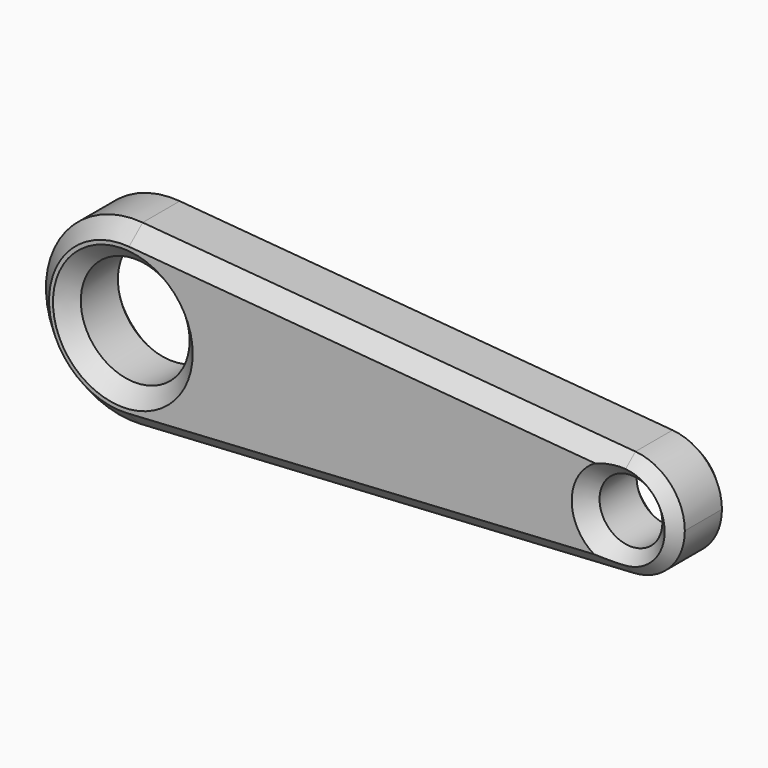
from build123d import *

# Parameters (mm, degrees)
F0_R         = 17.8816960504
F0_R_2       = 10.3302818728
F1_DEPTH     = 25.4
F2_T1_DEPTH  = 162.5438125483
F2_T3_DEPTH  = 162.5438125483
F2_T6_ANGLE  = 188.1812058846
F2_T8_ANGLE  = 171.8187941154
F2_T10_ANGLE = 188.1812058846
F2_T12_ANGLE = 171.8187941154


# Not quite as in the source:
# - a fillet or chamfer that OpenCascade refuses, or shapes differently, is made with other operations: its cross-section is extruded or revolved along the edge and cut away or added


with BuildPart() as f1:
    # F0 (on Front) → F1 (new body)
    with BuildSketch(Plane.XZ):
        with BuildLine():
            ThreePointArc((-128.3244462029, -9.9682561267), (-108.7150059464, -0.8082782893), (-100.7286188282, 19.3077094309))
            ThreePointArc((-100.7286188282, 19.3077094309), (-108.4686726557, 39.1591179408), (-127.6033017493, 48.5321015922))
            ThreePointArc((-127.6033017493, 48.5321015922), (-159.38061509, 19.669202563), (-128.3244462029, -9.9682561267))
        make_face()
        with Locations((-130.0557309645, 19.3077094309)):
            Circle(F0_R, mode=Mode.SUBTRACT)
        with BuildLine():
            ThreePointArc((-127.6033017493, 48.5321015922), (-108.4686726557, 39.1591179408), (-100.7286188282, 19.3077094309))
            ThreePointArc((-100.7286188282, 19.3077094309), (-108.7150059464, -0.8082782893), (-128.3244462029, -9.9682561267))
            Line((-128.3244462029, -9.9682561267), (33.9358894089, -0.3727110744))
            ThreePointArc((33.9358894089, -0.3727110744), (15.1895627408, 17.5172445164), (34.3711913147, 34.9396553669))
            Line((34.3711913147, 34.9396553669), (-127.6033017493, 48.5321015922))
        make_face()
        with BuildLine():
            ThreePointArc((50.5934622257, 17.2990376807), (45.9213605892, 29.2818740087), (34.3711913147, 34.9396553669))
            ThreePointArc((34.3711913147, 34.9396553669), (15.1895627408, 17.5172445164), (33.9358894089, -0.3727110744))
            ThreePointArc((33.9358894089, -0.3727110744), (45.772667286, 5.1564943288), (50.5934622257, 17.2990376807))
        make_face()
        with Locations((32.89084004, 17.2990376807)):
            Circle(F0_R_2, mode=Mode.SUBTRACT)
    extrude(amount=F1_DEPTH)

    # F2: chamfer of 5.08 on 12 edges, made by hand

    # F2_s2 → F2_t1 (cut)
    with BuildSketch(Plane(origin=(31.219303845, 0, -2.6198366217), x_dir=(0, 1, 0), z_dir=(-0.9964974398, 0, 0.0836232768))):
        Polygon((-20.32, -37.691508766), (-25.4, -32.611508766), (-25.4, -37.691508766), align=None)
        Polygon((-5.08, -37.691508766), (0, -32.611508766), (0, -37.691508766), align=None)
    extrude(amount=F2_T1_DEPTH, mode=Mode.SUBTRACT)

    # F2_s4 → F2_t3 (cut)
    with BuildSketch(Plane(origin=(-128.4646756887, 0, -7.5969803622), x_dir=(0, 1, 0), z_dir=(0.9982559968, 0, 0.0590335916))):
        Polygon((-20.32, -2.3754185022), (-25.4, 2.7045814978), (-25.4, -2.3754185022), align=None)
        Polygon((-5.08, -2.3754185022), (0, 2.7045814978), (0, -2.3754185022), align=None)
    extrude(amount=F2_T3_DEPTH, mode=Mode.SUBTRACT)

    # F2_s5 → F2_t6 (revolve, cut)
    with BuildSketch(Plane(origin=(-130.755189219, 0, 10.9726096036), x_dir=(0, 1, 0), z_dir=(0.9964974398, 0, -0.0836232768))):
        Polygon((-20.32, 37.691508766), (-25.4, 32.611508766), (-25.4, 37.691508766), align=None)
    revolve(axis=Axis((-130.0557309645, -25.4, 19.3077094309), (0, -1, 0)), revolution_arc=F2_T6_ANGLE, mode=Mode.SUBTRACT)

    # F2_s7 → F2_t8 (revolve, cut)
    with BuildSketch(Plane(origin=(33.7956599231, 0, 1.9985646901), x_dir=(0, 1, 0), z_dir=(-0.9982559968, 0, -0.0590335916))):
        Polygon((-20.32, 2.3754185022), (-25.4, -2.7045814978), (-25.4, 2.3754185022), align=None)
    revolve(axis=Axis((32.89084004, -25.4, 17.2990376807), (0, -1, 0)), revolution_arc=F2_T8_ANGLE, mode=Mode.SUBTRACT)

    # F2_s9 → F2_t10 (revolve, cut)
    with BuildSketch(Plane(origin=(-130.755189219, 0, 10.9726096036), x_dir=(0, 1, 0), z_dir=(0.9964974398, 0, -0.0836232768))):
        Polygon((-5.08, 37.691508766), (0, 32.611508766), (0, 37.691508766), align=None)
    revolve(axis=Axis((-130.0557309645, 0, 19.3077094309), (0, -1, 0)), revolution_arc=F2_T10_ANGLE, mode=Mode.SUBTRACT)

    # F2_s11 → F2_t12 (revolve, cut)
    with BuildSketch(Plane(origin=(33.7956599231, 0, 1.9985646901), x_dir=(0, 1, 0), z_dir=(-0.9982559968, 0, -0.0590335916))):
        Polygon((-5.08, 2.3754185022), (0, -2.7045814978), (0, 2.3754185022), align=None)
    revolve(axis=Axis((32.89084004, 0, 17.2990376807), (0, -1, 0)), revolution_arc=F2_T12_ANGLE, mode=Mode.SUBTRACT)

    # F2_s13 → F2_t14 (revolve, cut)
    with BuildSketch(Plane.XY.offset(19.3077094309)):
        Polygon((-112.1740349142, -5.08), (-107.0940349142, 0), (-112.1740349142, 0), align=None)
    revolve(axis=Axis((-130.0557309645, 0, 19.3077094309), (0, -1, 0)), mode=Mode.SUBTRACT)

    # F2_s15 → F2_t16 (revolve, cut)
    with BuildSketch(Plane.XY.offset(19.3077094309)):
        Polygon((-112.1740349142, -20.32), (-107.0940349142, -25.4), (-112.1740349142, -25.4), align=None)
    revolve(axis=Axis((-130.0557309645, -25.4, 19.3077094309), (0, -1, 0)), mode=Mode.SUBTRACT)

    # F2_s17 → F2_t18 (revolve, cut)
    with BuildSketch(Plane.XY.offset(17.2990376807)):
        Polygon((43.2211219128, -20.32), (48.3011219128, -25.4), (43.2211219128, -25.4), align=None)
    revolve(axis=Axis((32.89084004, -25.4, 17.2990376807), (0, -1, 0)), mode=Mode.SUBTRACT)

    # F2_s19 → F2_t20 (revolve, cut)
    with BuildSketch(Plane.XY.offset(17.2990376807)):
        Polygon((43.2211219128, -5.08), (48.3011219128, 0), (43.2211219128, 0), align=None)
    revolve(axis=Axis((32.89084004, 0, 17.2990376807), (0, -1, 0)), mode=Mode.SUBTRACT)


solid = f1.part
